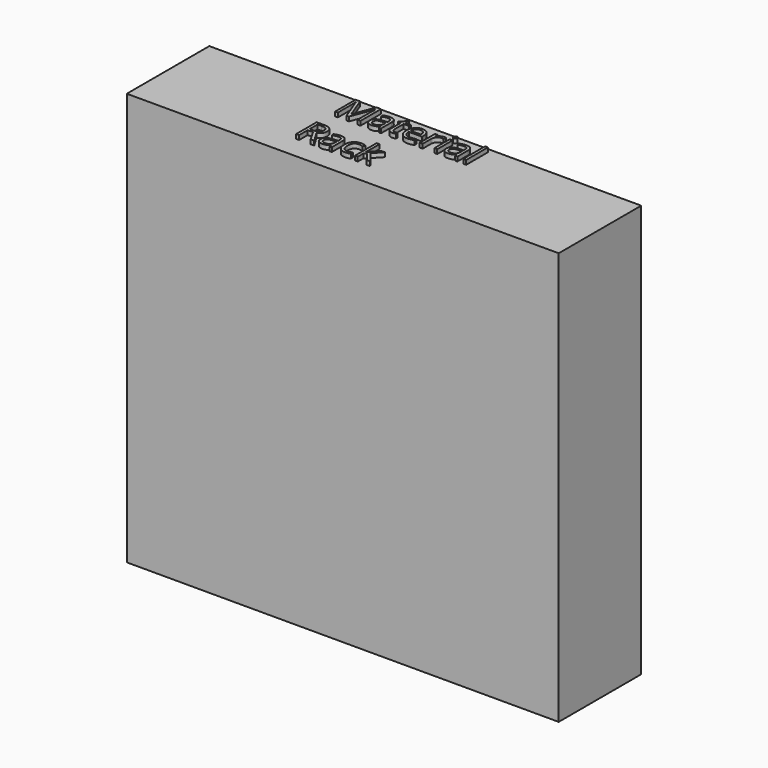
from build123d import *

# Parameters (mm, degrees)
F0_W         = 2552.7
F0_H         = 2438.4
F1_DEPTH     = 609.6
F2_TEXT_SIZE = 211.6666666667
F3_DEPTH     = 25.4


# Not quite as in the source:
# - Text() gives the source's letters only with a copy of the font that has no kerning and outlines rounded to 1/6400 em; it was checked with that copy


with BuildPart() as f1:
    # F0 (on Front) → F1 (new body)
    with BuildSketch(Plane.XZ):
        Rectangle(F0_W, F0_H)
    extrude(amount=F1_DEPTH)

    # F2 (on face) → F3 (join)
    with BuildSketch(Plane.XY.offset(1219.2)):
        with Locations((-404.51484375, -185.8439427276)):
            Text('Material', F2_TEXT_SIZE, font='Open Sans', text_align=(TextAlign.LEFT, TextAlign.BOTTOM))
        with Locations((-404.51484375, -473.7106093943)):
            Text('Rack', F2_TEXT_SIZE, font='Open Sans', text_align=(TextAlign.LEFT, TextAlign.BOTTOM))
    extrude(amount=F3_DEPTH)


solid = f1.part
